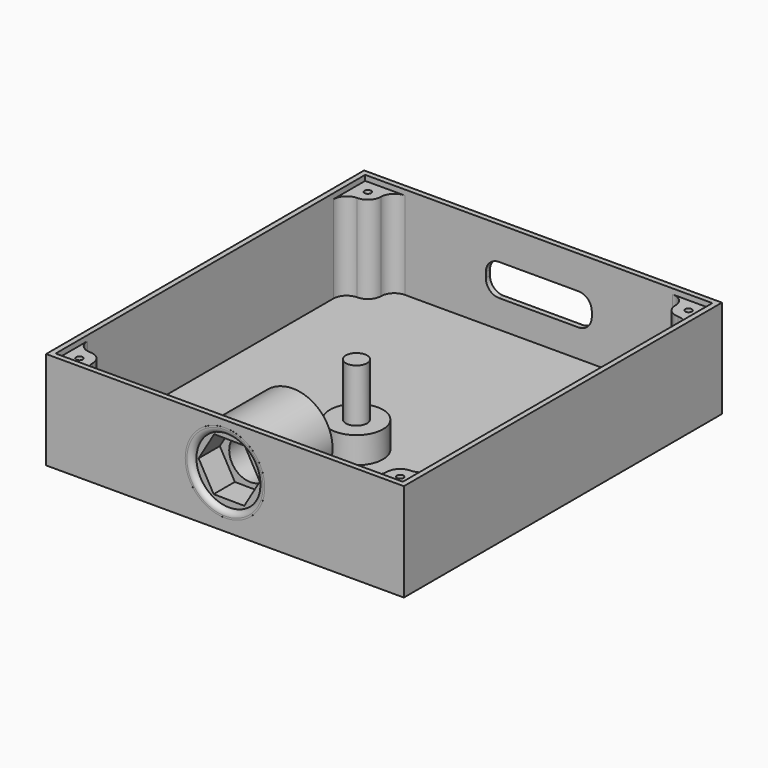
from build123d import *

# Parameters (mm, degrees)
F0_W      = 135
F0_H      = 150
F1_DEPTH  = 2
F2_W      = 135
F2_H      = 150
F2_W_2    = 131
F2_H_2    = 146
F3_DEPTH  = 35
F4_R      = 4
F5_DEPTH  = 30
F6_R      = 10
F6_R_2    = 4
F7_DEPTH  = 10
F9_R      = 15
F10_DEPTH = 10
F8_R      = 15
F12_DEPTH = 5
F13_R     = 15
F13_R_2   = 8
F14_DEPTH = 20
F15_W     = 40
F15_H     = 12
F16_DEPTH = 2
F17_R     = 5
F18_W     = 10
F18_H     = 10
F19_DEPTH = 33
F20_R     = 1.25
F21_DEPTH = 35.001
F22_R     = 4.99999
F23_R     = 12.3556147712
F24_DEPTH = 2
F25_R     = 1.99999


# Not quite as in the source:
# - a fillet or chamfer is up to 0.001 mm smaller than in the source, because OpenCascade refuses the exact size
# - ends of sketch curves that miss each other by under 0.0002 mm in the source are joined
# - a feature of the source that left no trace in its solid (it failed there, or was rolled back) is left out


with BuildPart() as f1:
    # F0 (on Top) → F1 (new body)
    with BuildSketch(Plane.XY):
        Rectangle(F0_W, F0_H)
    extrude(amount=F1_DEPTH)

    # F2 (on face) → F3 (join)
    with BuildSketch(Plane.XY.offset(2)):
        Rectangle(F2_W, F2_H)
        Rectangle(F2_W_2, F2_H_2, mode=Mode.SUBTRACT)
    extrude(amount=F3_DEPTH)

    # F4 (on face) → F5 (join)
    with BuildSketch(Plane.XY.offset(2)):
        with Locations((0, -13)):
            Circle(F4_R)
    extrude(amount=F5_DEPTH)

    # F6 (on face) → F7 (join)
    with BuildSketch(Plane.XY.offset(2)):
        with Locations((0, -13)):
            Circle(F6_R)
        with Locations((0, -13)):
            Circle(F6_R_2, mode=Mode.SUBTRACT)
    extrude(amount=F7_DEPTH)

    # F8 (on face) → F12 (cut)
    with BuildSketch(Plane(origin=(0, -73, 0), x_dir=(-1, 0, 0), z_dir=(0, 1, 0))):
        with Locations((0, 19.5)):
            Circle(F8_R)
    extrude(amount=-F12_DEPTH, mode=Mode.SUBTRACT)

    # F15 (on face) → F16 (cut)
    with BuildSketch(Plane(origin=(0, 75, 0), x_dir=(-1, 0, 0), z_dir=(0, 1, 0))):
        with Locations((0, 18.5)):
            Rectangle(F15_W, F15_H)
    extrude(amount=-F16_DEPTH, mode=Mode.SUBTRACT)

    # F17
    f17_edges = [f1.edges().sort_by_distance(p)[0] for p in [
        (-20, 74, 12.5),
        (20, 74, 12.5),
        (-20, 74, 24.5),
        (20, 74, 24.5),
    ]]
    fillet(f17_edges, radius=F17_R)

    # F18 (on face) → F19 (join)
    with BuildSketch(Plane.XY.offset(2)):
        with Locations((-60.5, 68)):
            Rectangle(F18_W, F18_H)
        with Locations((60.5, 68)):
            Rectangle(F18_W, F18_H)
        with Locations((60.5, -68)):
            Rectangle(F18_W, F18_H)
        with Locations((-60.5, -68)):
            Rectangle(F18_W, F18_H)
    extrude(amount=F19_DEPTH)

    # F20 (on face) → F21 (cut, through all)
    with BuildSketch(Plane.XY.offset(35)):
        with Locations((-60.5, 68)):
            Circle(F20_R)
        with Locations((60.5, 68)):
            Circle(F20_R)
        with Locations((60.5, -68)):
            Circle(F20_R)
        with Locations((-60.5, -68)):
            Circle(F20_R)
    extrude(amount=-F21_DEPTH, mode=Mode.SUBTRACT)

    # F22 (radius 5 in the source; OpenCascade refuses exactly that, so slightly less here)
    f22_edges = [f1.edges().sort_by_distance(p)[0] for p in [
        (-55.5, 73, 18.5),
        (-55.5, 63, 18.5),
        (-65.5, 63, 18.5),
        (55.5, 73, 18.5),
        (55.5, 63, 18.5),
        (65.5, 63, 18.5),
        (65.5, -63, 18.5),
        (55.5, -63, 18.5),
        (55.5, -73, 18.5),
        (-65.5, -63, 18.5),
        (-55.5, -63, 18.5),
        (-55.5, -73, 18.5),
    ]]
    fillet(f22_edges, radius=F22_R)


with BuildPart() as f10:
    # F9 (on face) → F10 (new body)
    with BuildSketch(Plane(origin=(0, -73, 0), x_dir=(-1, 0, 0), z_dir=(0, 1, 0))):
        with Locations((0, 19.5)):
            Circle(F9_R)
        Polygon((5.6714946114, 29.6733575716), (11.5464081104, 19.7325968002), (5.874913499, 9.6743920794), (-5.6714946114, 9.5569481299), (-11.5464081104, 19.4977089013), (-5.874913499, 29.5559136221), align=None, mode=Mode.SUBTRACT)
    extrude(amount=F10_DEPTH)

    # F13 (on face) → F14 (join)
    with BuildSketch(Plane(origin=(0, -63, 0), x_dir=(-1, 0, 0), z_dir=(0, 1, 0))):
        with Locations((0, 19.5)):
            Circle(F13_R)
        Polygon((-5.874913499, 29.5559136221), (5.6714946114, 29.6733575716), (11.5464081104, 19.7325968002), (5.874913499, 9.6743920794), (-5.6714946114, 9.5569481299), (-11.5464081104, 19.4977089013), align=None, mode=Mode.SUBTRACT)
        Polygon((11.5464081104, 19.7325968002), (5.6714946114, 29.6733575716), (-5.874913499, 29.5559136221), (-11.5464081104, 19.4977089013), (-5.6714946114, 9.5569481299), (5.874913499, 9.6743920794), align=None)
        with Locations((0, 19.5)):
            Circle(F13_R_2, mode=Mode.SUBTRACT)
    extrude(amount=F14_DEPTH)


with BuildPart() as f24:
    # F23 (on face) → F24 (new body)
    with BuildSketch(Plane(origin=(0, -73, 0), x_dir=(-1, 0, 0), z_dir=(0, 1, 0))):
        with BuildLine():
            ThreePointArc((-14.9999967303, 19.4900959839), (-0.0049520018, 4.5000008174), (14.9999869214, 19.4801919852))
            ThreePointArc((14.9999869214, 19.4801919852), (14.9999967304, 19.4900959775), (14.9999869214, 19.4999999827))
            ThreePointArc((14.9999869214, 19.4999999827), (-0.0049520018, 34.4801911505), (-14.9999967303, 19.4900959839))
        make_face()
        with Locations((0, 19.4801919679)):
            Circle(F23_R, mode=Mode.SUBTRACT)
    extrude(amount=-F24_DEPTH)

    # F25 (radius 2 in the source; OpenCascade refuses exactly that, so slightly less here)
    f25_edges = [f24.edges().sort_by_distance(p)[0] for p in [
        (12.355615, -75, 19.480192),
    ]]
    fillet(f25_edges, radius=F25_R)


solid = Compound([f1.part, f10.part, f24.part])
